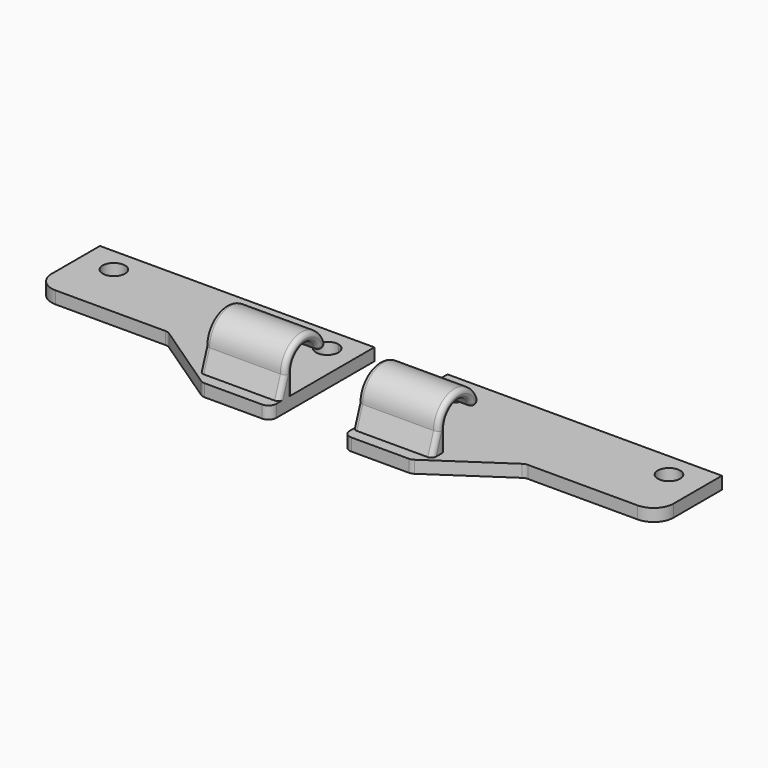
from build123d import *

# Parameters (mm, degrees)
F0_R      = 2.8
F1_DEPTH  = 3.1
F2_W      = 20
F2_H      = 2.3
F3_DEPTH  = 5.1
F3_FACE_W = 20
F3_FACE_H = 2.3
F5_ANGLE  = 170
F6_R      = 1.14999
F8_DEPTH  = 20
F9_R      = 1.14


# Not quite as in the source:
# - a fillet or chamfer is up to 0.001 mm smaller than in the source, because OpenCascade refuses the exact size
# - ends of sketch curves that miss each other by under 0.0002 mm in the source are joined


with BuildPart() as f1:
    # F0 (on Top) → F1 (new body)
    with BuildSketch(Plane.XY):
        with BuildLine():
            Line((37.938385576, 27.4999964178), (36.738385576, 27.4999964178))
            Line((36.738385576, 27.4999964178), (-20.7205781263, 27.4999964178))
            Line((-20.7205781263, 27.4999964178), (-25.7205781263, 27.4999966308))
            Line((-25.7205781263, 27.4999966308), (-25.7205781263, 22.4999966308))
            Line((-25.7205781263, 22.4999966308), (-25.7205781263, 12.3999966308))
            ThreePointArc((-25.7205781263, 12.3999966308), (-24.2561120322, 8.8644627249), (-20.7205781263, 7.3999966308))
            Line((-20.7205781263, 7.3999966308), (6.7794218737, 7.3999964178))
            ThreePointArc((6.7794218737, 7.3999964178), (7.3637845142, 7.312722301), (7.8971474214, 7.0585167222))
            Line((7.8971474214, 7.0585167222), (25.4316860469, -4.7585238867))
            ThreePointArc((25.4316860469, -4.7585238867), (25.9650489541, -5.0127294655), (26.5494115945, -5.1000035822))
            Line((26.5494115945, -5.1000035822), (40.938385576, -5.1000035822))
            ThreePointArc((40.938385576, -5.1000035822), (42.3525991384, -4.5142171446), (42.938385576, -3.1000035822))
            Line((42.938385576, -3.1000035822), (42.938385576, 7.3999964178))
            Line((42.938385576, 7.3999964178), (42.938385576, 22.4999964178))
            Line((42.938385576, 22.4999964178), (42.938385576, 27.4999964178))
            Line((42.938385576, 27.4999964178), (37.938385576, 27.4999964178))
        make_face()
        with Locations((-17.351614424, 21.3999971747)):
            Circle(F0_R, mode=Mode.SUBTRACT)
        with BuildLine():
            ThreePointArc((38.838385576, 21.3999964178), (33.8247912139, 19.6853535978), (36.738385576, 24.1110847601))
            ThreePointArc((36.738385576, 24.1110847601), (38.2519799381, 23.1146392377), (38.838385576, 21.3999964178))
        make_face(mode=Mode.SUBTRACT)
    extrude(amount=F1_DEPTH)

    # F2 (on face) → F3 (join)
    with BuildSketch(Plane.XY.offset(3.1)):
        with Locations((32.938385576, 0.6874617912)):
            Rectangle(F2_W, F2_H)
    extrude(amount=F3_DEPTH)

    # F3_face (on face) → F5 (revolve)
    with BuildSketch(Plane(origin=(32.938385576, 0.6874617912, 8.2), x_dir=(1, 0, 0), z_dir=(0, 0, 1))):
        Rectangle(F3_FACE_W, F3_FACE_H)
    revolve(axis=Axis((32.938385576, 6.1304703801, 8.2), (-1, 0, 0)), revolution_arc=F5_ANGLE)

    # F6 (radius 1.15 in the source; OpenCascade refuses exactly that, so slightly less here)
    f6_edges = [f1.edges().sort_by_distance(p)[0] for p in [
        (32.938386, 10.358259, 8.945473),
        (32.938386, 12.623316, 9.344864),
    ]]
    fillet(f6_edges, radius=F6_R)

    # F7 (on face) → F8 (join)
    with BuildSketch(Plane(origin=(22.938385576, 0, 0), x_dir=(0, -1, 0), z_dir=(-1, 0, 0))):
        Polygon((2.2625382088, 3.1), (0.4625382088, 8.2), (0.4625382088, 3.1), align=None)
    extrude(amount=-F8_DEPTH)

    # F9
    f9_edges = [f1.edges().sort_by_distance(p)[0] for p in [
        (22.938386, -1.362538, 5.65),
        (22.938386, 4.861326, 14.669701),
        (42.938386, -1.362538, 5.65),
        (42.938386, 4.861326, 14.669701),
    ]]
    fillet(f9_edges, radius=F9_R)


with BuildPart() as f1_1:
    # F10: moved
    add(f1.part.moved(Location((-52.1, 0, 0))))


with BuildPart() as f11_1:
    # F11: instance of F1
    add(f1_1.part.mirror(Plane.YZ))


solid = Compound([f1_1.part, f11_1.part])
